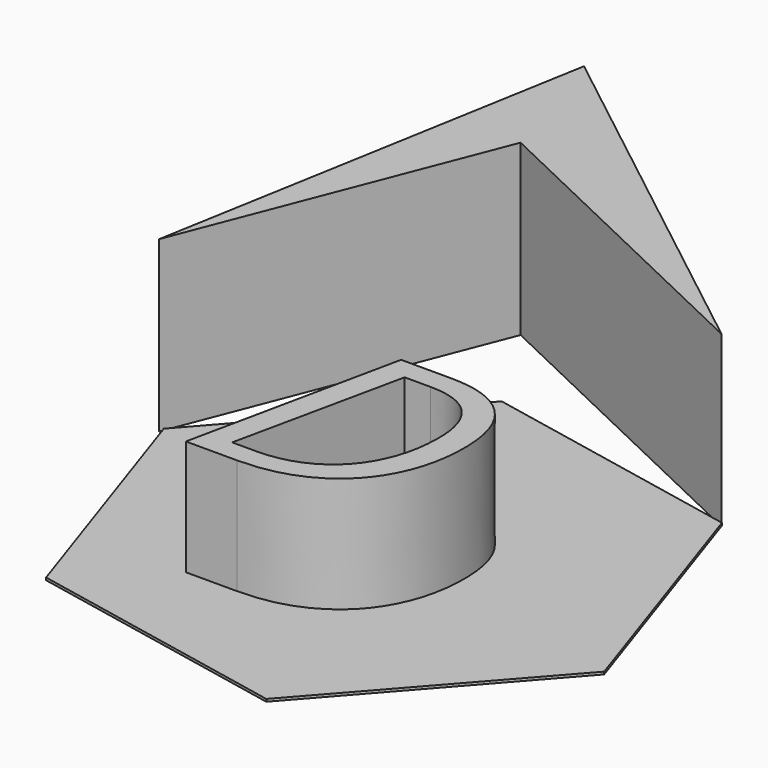
from build123d import *

# Parameters (mm, degrees)
F1_DEPTH     = 0.3
F3_DEPTH     = 20
F4_DEPTH     = 13.9
F5_DEPTH     = 20.3
F6_DEPTH     = 16.6
F7_DEPTH     = 6.6
F8_R         = 3.6699379177
F8_TEXT_SIZE = 35.7302367128
F9_DEPTH     = 14.1


# Not quite as in the source:
# - a feature of the source that left no trace in its solid (it failed there, or was rolled back) is left out
# - Text() gives the source's letters only with a copy of the font that has no kerning and outlines rounded to 1/6400 em; it was checked with that copy


with BuildPart() as f1:
    # F0 (on Top) → F1 (new body)
    with BuildSketch(Plane.XY):
        Polygon((-31.4685011597, 6.3512263582), (-21.2345739512, -24.0769082442), (10.2339272085, -30.4281346024), (31.4685011597, -6.3512263582), (21.2345739512, 24.0769082442), (-10.2339272085, 30.4281346024), align=None)
    extrude(amount=F1_DEPTH)


with BuildPart() as f3:
    # F2 (on Top) → F3 (new body)
    with BuildSketch(Plane.XY):
        Polygon((-23.0069048703, 58.7191171944), (-32.1638807654, 6.5243463032), (-17.9705675691, 42.9233312607), (20.9465865046, 24.3804510683), align=None)
    extrude(amount=F3_DEPTH)

    # F4 (add): a face of the model
    f4_faces = [f3.faces().sort_by_distance(p)[0] for p in [
        (-1.4885976843, 40.9629828664, 20),
    ]]
    extrude(f4_faces, amount=-F4_DEPTH)

    # F5 (add): a face of the model
    f5_faces = [f3.faces().sort_by_distance(p)[0] for p in [
        (-1.4885976843, 40.9629828664, 20),
    ]]
    extrude(f5_faces, amount=-F5_DEPTH)

    # F6 (add): a face of the model
    f6_faces = [f3.faces().sort_by_distance(p)[0] for p in [
        (-1.4885976843, 40.9629828664, 20),
    ]]
    extrude(f6_faces, amount=-F6_DEPTH)

    # F7 (add): a face of the model
    f7_faces = [f3.faces().sort_by_distance(p)[0] for p in [
        (-1.4885976843, 40.9629828664, 20),
    ]]
    extrude(f7_faces, amount=-F7_DEPTH)


with BuildPart() as f9:
    # F8 (on Top) → F9 (new body)
    with BuildSketch(Plane.XY):
        with Locations((-20.0308859348, 50.4778362811)):
            Circle(F8_R)
        with Locations((-13.1804875346, -15.0861003522)):
            Text('D', F8_TEXT_SIZE, font='Open Sans', font_style=FontStyle.ITALIC, text_align=(TextAlign.LEFT, TextAlign.BOTTOM))
    extrude(amount=F9_DEPTH)


solid = Compound([f1.part, f3.part, f9.part])
